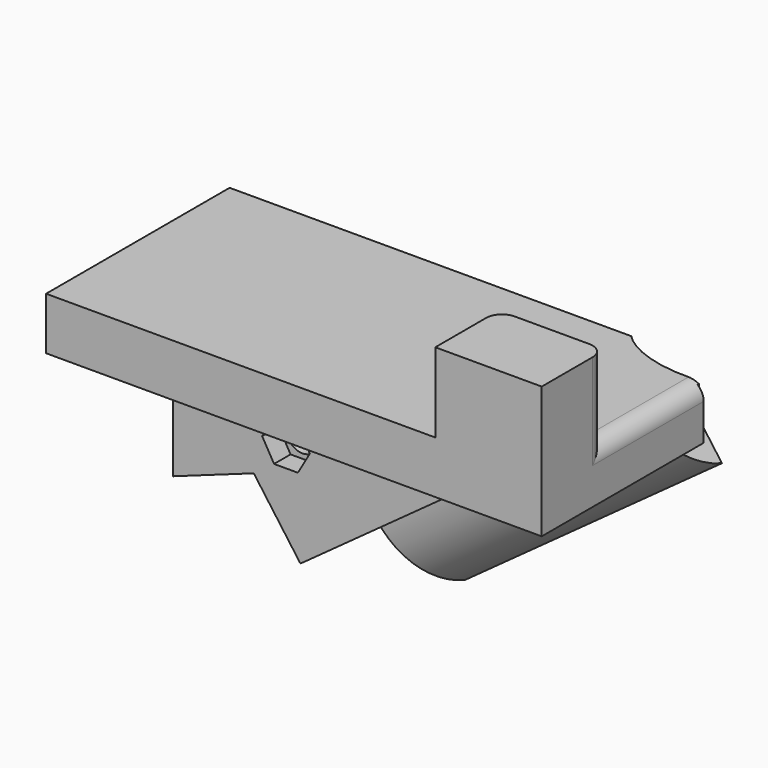
from build123d import *
from build123d import SkipClean  # not in build123d's __all__

# Parameters (mm, degrees)
F0_W      = 131
F0_H      = 155.25
F0_R      = 5
F0_R_2    = 10
F1_DEPTH  = 12.7
F2_DEPTH  = 150
F3_R      = 4.7625
F4_DEPTH  = 167.951
F6_DEPTH  = 55
F9_W      = 46.4503765106
F9_H      = 23.6088857055
F10_DEPTH = 100.6187200546
F12_DEPTH = 150.001
F14_DEPTH = 89.0000760555
F15_R     = 16
F16_DEPTH = 210.4837932836
F18_W     = 28.0103459954
F18_H     = 33.3821959794
F19_DEPTH = 57.4413500726
F23_DEPTH = 37.3063087463
F25_DEPTH = 262.8513174901
F26_W     = 130
F26_H     = 33
F27_DEPTH = 25
F28_DEPTH = 47.1665114164
F29_W     = 130
F29_H     = 16.5
F30_DEPTH = 118.0664598942
F32_DEPTH = 6.5
F33_R     = 5
F34_DEPTH = 47.2060309181
F35_W     = 63.7330800295
F35_H     = 16.5
F36_DEPTH = 26
F37_W     = 33.5
F37_H     = 25
F38_DEPTH = 25
F39_R     = 5
F41_DEPTH = 150.837957859


with BuildPart() as f1:
    # F0 (on Front) → F1 (new body)
    with BuildSketch(Plane.XZ):
        with Locations((0, 77.625)):
            Rectangle(F0_W, F0_H)
        with Locations((-32.75, 57)):
            Circle(F0_R, mode=Mode.SUBTRACT)
        with Locations((32.75, 57)):
            Circle(F0_R, mode=Mode.SUBTRACT)
        with Locations((0, 89.75)):
            Circle(F0_R_2, mode=Mode.SUBTRACT)
        with Locations((-32.75, 122.5)):
            Circle(F0_R, mode=Mode.SUBTRACT)
        with Locations((32.75, 122.5)):
            Circle(F0_R, mode=Mode.SUBTRACT)
    extrude(amount=-F1_DEPTH)

    # F0 (on Front) → F2 (join)
    with BuildSketch(Plane.XZ):
        Polygon((89.5, 0), (65.5, 0), (-65.5, 0), (-65.5, -12.7), (89.5, -12.7), align=None)
    extrude(amount=-F2_DEPTH)

    # F3 (on face) → F4 (cut, through all)
    with BuildSketch(Plane(origin=(0, 0, -12.7), x_dir=(1, 0, 0), z_dir=(0, 0, -1))):
        with Locations((-40, -55.7)):
            Circle(F3_R)
        with Locations((-40, -118.2)):
            Circle(F3_R)
        with Locations((64, -118.2)):
            Circle(F3_R)
        with Locations((64, -55.7)):
            Circle(F3_R)
    extrude(amount=-F4_DEPTH, mode=Mode.SUBTRACT)

    # F5 (on face) → F6 (join)
    with BuildSketch(Plane.XZ):
        Polygon((76.5, -12.7), (-63.5, -12.7), (-44.9285714286, -100.7630571853), align=None)
    extrude(amount=-F6_DEPTH)

    # F7 (on face) → F8 (revolve)
    with BuildSketch(Plane(origin=(32.4031609217, 0, -44.6801379177), x_dir=(0.8095238095, 0, 0.5870870479), z_dir=(0.5870870479, 0, -0.8095238095))):
        Polygon((18.2698592544, -40), (54.4725659202, -40), (54.4725659202, -30), (-45.5274340798, -30), (-45.5274340798, -40), align=None)
    revolve(axis=Axis((36.0238095238, 55, -42.0543523951), (-0.8095238095, 0, -0.5870870479)))

    # F9 (on face) → F10 (cut)
    with BuildSketch(Plane.YZ.offset(89.5)):
        with Locations((57.3695674539, 11.8044428527)):
            Rectangle(F9_W, F9_H)
    extrude(amount=-F10_DEPTH, mode=Mode.SUBTRACT)

    # F11 (on Front) → F12 (cut, through all)
    with BuildSketch(Plane.XZ):
        Polygon((-55.6169226766, -72.8361010551), (-44.6262694895, -72.8361010551), (-44.6262694895, -12.6905664802), (-63.8953074813, -12.6905664802), (-63.8953074813, -72.8361010551), align=None)
        Polygon((-4.5890193433, -104.113265872), (-4.5890193433, -72.8361010551), (-44.6262694895, -72.8361010551), (-55.6169226766, -72.8361010551), (-55.6169226766, -104.113265872), align=None)
    extrude(amount=-F12_DEPTH, mode=Mode.SUBTRACT)

    # F13 (on face) → F14 (cut)
    with BuildSketch(Plane(origin=(0, 55, 0), x_dir=(-1, 0, 0), z_dir=(0, 1, 0))):
        Polygon((76.3912552581, -71.6465198879), (44.6262694895, -60.2878452083), (44.6262694895, -72.8361010551), (6.4205920826, -72.8361010551), (4.4523809524, -71.4087047902), (-10.0519139283, -91.4084170785), (37.2047263411, -125.6801223738), align=None)
        Polygon((44.6262694895, -60.2878452083), (19.1295571499, -51.1706095521), (13.2586866709, -59.2658476473), (4.4523809524, -71.4087047902), (6.4205920826, -72.8361010551), (44.6262694895, -72.8361010551), align=None)
    extrude(amount=-F14_DEPTH, mode=Mode.SUBTRACT)

    # F15 (on face) → F16 (cut, through all)
    with BuildSketch(Plane(origin=(-36.8555418741, 0, -26.7285668724), x_dir=(0, -1, 0), z_dir=(-0.8095238095, 0, -0.5870870479))):
        with Locations((-55, -55.1931115454)):
            Circle(F15_R)
        with BuildLine():
            ThreePointArc((-40, -55.1931115454), (-65.6066017178, -65.7997132632), (-55, -40.1931115454))
            Line((-55, -40.1931115454), (-55, -55.1931115454))
            Line((-55, -55.1931115454), (-40, -55.1931115454))
        make_face(mode=Mode.SUBTRACT)
        with BuildLine():
            Line((-55, -55.1931115454), (-55, -40.1931115454))
            ThreePointArc((-55, -40.1931115454), (-65.6066017178, -65.7997132632), (-40, -55.1931115454))
            Line((-40, -55.1931115454), (-55, -55.1931115454))
        make_face()
    with SkipClean():  # cleaning this boolean's faces spoils the solid; the shape is the same uncleaned
        extrude(amount=-F16_DEPTH, mode=Mode.SUBTRACT)

    # F18 (on offset) → F19 (cut)
    with BuildSketch(Plane(origin=(0, 0, -69.7121929049), x_dir=(1, 0, 0), z_dir=(0, 0, -1))):
        with Locations((-40.2482412755, -55.8588486165)):
            Rectangle(F18_W, F18_H)
    with SkipClean():  # cleaning this boolean's faces spoils the solid; the shape is the same uncleaned
        extrude(amount=-F19_DEPTH, mode=Mode.SUBTRACT)

    # F22 (on offset) → F23 (join)
    with BuildSketch(Plane(origin=(0, 66.3563400507, 0), x_dir=(-1, 0, 0), z_dir=(0, 1, 0))):
        Polygon((-19.5, -25.368578732), (9.2864632607, -47.1396760544), (25.5, -47.1396760544), (25.5, -10.8354373375), (-19.5, -10.8354373375), align=None)
    with SkipClean():  # cleaning this boolean's faces spoils the solid; the shape is the same uncleaned
        extrude(amount=-F23_DEPTH)

    # F24 (on offset) → F25 (cut, through all)
    with BuildSketch(Plane(origin=(0, 0, -107.6003174901), x_dir=(1, 0, 0), z_dir=(0, 0, -1))):
        Polygon((105.054743588, -47.2050309181), (-70.2532827854, -47.2050309181), (-70.2532827854, -164.4858419895), (108.5324063897, -164.4858419895), align=None)
    extrude(amount=-F25_DEPTH, mode=Mode.SUBTRACT)

    # F26 (on Front) → F27 (join)
    with BuildSketch(Plane.XZ):
        with Locations((0.4943662184, -6)):
            Rectangle(F26_W, F26_H)
    extrude(amount=F27_DEPTH)

    # F28 (add): a face of the model
    f28_faces = [f1.faces().sort_by_distance(p)[0] for p in [
        (-54.5656671683, 0, -17.5954279167),
    ]]
    extrude(f28_faces, amount=F28_DEPTH)

    # F29 (on face) → F30 (cut)
    with BuildSketch(Plane.XZ.offset(25)):
        Polygon((65.4943662184, -6), (102.4388783057, -6), (114.364810288, 171.1933612823), (-95.0750373681, 171.1933612823), (-95.0750373681, -6), (-64.5056337816, -6), (-64.5056337816, 10.5), (65.4943662184, 10.5), align=None)
        with Locations((0.4943662184, 2.25)):
            Rectangle(F29_W, F29_H)
    extrude(amount=-F30_DEPTH, mode=Mode.SUBTRACT)

    # F31 (on face) → F32 (cut)
    with BuildSketch(Plane.XZ):
        Polygon((-12.7527767497, -46.5), (-5.2472232503, -46.5), (-1.4944465005, -40), (-5.2472232503, -33.5), (-12.7527767497, -33.5), (-16.5055534995, -40), align=None)
    extrude(amount=-F32_DEPTH, mode=Mode.SUBTRACT)

    # F33 (on face) → F34 (cut, through all)
    with BuildSketch(Plane.XZ):
        with Locations((-9, -40)):
            Circle(F33_R)
    extrude(amount=-F34_DEPTH, mode=Mode.SUBTRACT)

    # F35 (on face) → F36 (join)
    with BuildSketch(Plane.YZ.offset(65.4943662184)):
        with Locations((6.8665400147, -14.25)):
            Rectangle(F35_W, F35_H)
    extrude(amount=F36_DEPTH)

    # F37 (on face) → F38 (join)
    with BuildSketch(Plane.XY.offset(-6)):
        with Locations((74.7443662184, -12.5)):
            Rectangle(F37_W, F37_H)
    extrude(amount=F38_DEPTH)

    # F39
    f39_edges = [f1.edges().sort_by_distance(p)[0] for p in [
        (57.994366, 0, 6.5),
        (91.494366, 0, 6.5),
        (91.494366, 19.36654, -6),
    ]]
    fillet(f39_edges, radius=F39_R)

    # F40 (on face) → F41 (cut)
    with BuildSketch(Plane(origin=(0, 0, -22.5), x_dir=(1, 0, 0), z_dir=(0, 0, -1))):
        Polygon((-64.5056337816, -47.1665114164), (-64.5056337816, 25), (-82.232825458, 25), (-82.232825458, -50.1768067479), (-64.5056337816, -50.1768067479), align=None)
    extrude(amount=-F41_DEPTH, mode=Mode.SUBTRACT)


solid = f1.part
